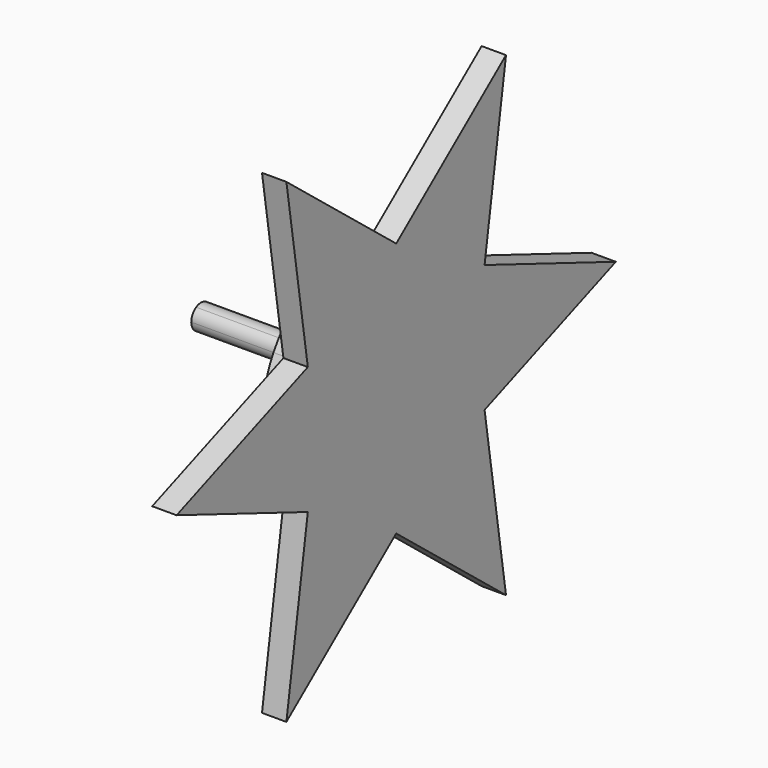
from build123d import *

# Parameters (mm, degrees)
F1_DEPTH = 40.64
F2_DEPTH = 10.16
F3_DEPTH = 5.08


with BuildPart() as f1:
    # F0 (on Right) → F1 (new body)
    with BuildSketch(Plane.YZ):
        with BuildLine():
            Line((-1.27, -2.1997045256), (0, 0))
            Line((0, 0), (-2.54, 0))
            ThreePointArc((-2.54, 0), (-2.1997045256, -1.27), (-1.27, -2.1997045256))
        make_face()
        with BuildLine():
            Line((1.27, -2.1997045256), (0, 0))
            Line((0, 0), (-1.27, -2.1997045256))
            ThreePointArc((-1.27, -2.1997045256), (0, -2.54), (1.27, -2.1997045256))
        make_face()
        with BuildLine():
            ThreePointArc((1.27, -2.1997045256), (2.1997045256, -1.27), (2.54, 0))
            Line((2.54, 0), (0, 0))
            Line((0, 0), (1.27, -2.1997045256))
        make_face()
        with BuildLine():
            Line((0, 0), (2.54, 0))
            ThreePointArc((2.54, 0), (2.1997045256, 1.27), (1.27, 2.1997045256))
            Line((1.27, 2.1997045256), (0, 0))
        make_face()
        with BuildLine():
            Line((-1.27, 2.1997045256), (0, 0))
            Line((0, 0), (1.27, 2.1997045256))
            ThreePointArc((1.27, 2.1997045256), (0, 2.54), (-1.27, 2.1997045256))
        make_face()
        with BuildLine():
            Line((-2.54, 0), (0, 0))
            Line((0, 0), (-1.27, 2.1997045256))
            ThreePointArc((-1.27, 2.1997045256), (-2.1997045256, 1.27), (-2.54, 0))
        make_face()
    extrude(amount=-F1_DEPTH)

    # F0 (on Right) → F2 (join)
    with BuildSketch(Plane.YZ):
        with BuildLine():
            ThreePointArc((21.6980938733, -4.8107532948), (22.0928807689, -2.419761214), (22.225, 0))
            Line((22.225, 0), (20.9576915714, 0))
            Line((20.9576915714, 0), (21.6980938733, -4.8107532948))
        make_face()
        with BuildLine():
            Line((20.9576915714, 0), (22.225, 0))
            ThreePointArc((22.225, 0), (22.0928807689, 2.4197612139), (21.6980938733, 4.8107532948))
            Line((21.6980938733, 4.8107532948), (20.9576915714, 0))
        make_face()
        with BuildLine():
            Line((19.2474145991, -11.1125), (20.9576915714, 0))
            Line((20.9576915714, 0), (2.54, 0))
            ThreePointArc((2.54, 0), (2.1997045256, -1.27), (1.27, -2.1997045256))
            Line((1.27, -2.1997045256), (10.4788457857, -18.1498933056))
            Line((10.4788457857, -18.1498933056), (19.2474145991, -11.1125))
        make_face()
        with BuildLine():
            Line((2.54, 0), (20.9576915714, 0))
            Line((20.9576915714, 0), (19.2474145991, 11.1125))
            Line((19.2474145991, 11.1125), (10.4788457857, 18.1498933056))
            Line((10.4788457857, 18.1498933056), (1.27, 2.1997045256))
            ThreePointArc((1.27, 2.1997045256), (2.1997045256, 1.27), (2.54, 0))
        make_face()
        with BuildLine():
            Line((19.2474145991, 11.1125), (20.9576915714, 0))
            Line((20.9576915714, 0), (21.6980938733, 4.8107532948))
            ThreePointArc((21.6980938733, 4.8107532948), (20.713803825, 8.0553681542), (19.2474145991, 11.1125))
        make_face()
        with BuildLine():
            Line((21.6980938733, -4.8107532948), (20.9576915714, 0))
            Line((20.9576915714, 0), (19.2474145991, -11.1125))
            ThreePointArc((19.2474145991, -11.1125), (20.713803825, -8.0553681542), (21.6980938733, -4.8107532948))
        make_face()
        with BuildLine():
            Line((10.4788457857, 18.1498933056), (11.1125, 19.2474145991))
            ThreePointArc((11.1125, 19.2474145991), (8.9508657021, 20.3428765956), (6.682812372, 21.1964771554))
            Line((6.682812372, 21.1964771554), (10.4788457857, 18.1498933056))
        make_face()
        with BuildLine():
            ThreePointArc((15.0152815013, 16.3857238606), (13.1420150668, 17.9231153816), (11.1125, 19.2474145991))
            Line((11.1125, 19.2474145991), (10.4788457857, 18.1498933056))
            Line((10.4788457857, 18.1498933056), (15.0152815013, 16.3857238606))
        make_face()
        with BuildLine():
            Line((10.4788457857, -18.1498933056), (11.1125, -19.2474145991))
            ThreePointArc((11.1125, -19.2474145991), (13.1420150668, -17.9231153816), (15.0152815013, -16.3857238606))
            Line((15.0152815013, -16.3857238606), (10.4788457857, -18.1498933056))
        make_face()
        with BuildLine():
            ThreePointArc((6.682812372, -21.1964771554), (8.9508657021, -20.3428765956), (11.1125, -19.2474145991))
            Line((11.1125, -19.2474145991), (10.4788457857, -18.1498933056))
            Line((10.4788457857, -18.1498933056), (6.682812372, -21.1964771554))
        make_face()
        with BuildLine():
            ThreePointArc((19.2474145991, 11.1125), (17.3330553708, 13.9109962444), (15.0152815013, 16.3857238606))
            Line((15.0152815013, 16.3857238606), (10.4788457857, 18.1498933056))
            Line((10.4788457857, 18.1498933056), (19.2474145991, 11.1125))
        make_face()
        with BuildLine():
            Line((10.4788457857, -18.1498933056), (15.0152815013, -16.3857238606))
            ThreePointArc((15.0152815013, -16.3857238606), (17.3330553708, -13.9109962444), (19.2474145991, -11.1125))
            Line((19.2474145991, -11.1125), (10.4788457857, -18.1498933056))
        make_face()
        with BuildLine():
            Line((-10.4788457857, 18.1498933056), (-11.1125, 19.2474145991))
            ThreePointArc((-11.1125, 19.2474145991), (-13.1420150668, 17.9231153816), (-15.0152815013, 16.3857238606))
            Line((-15.0152815013, 16.3857238606), (-10.4788457857, 18.1498933056))
        make_face()
        with BuildLine():
            ThreePointArc((-6.682812372, 21.1964771554), (-8.9508657021, 20.3428765956), (-11.1125, 19.2474145991))
            Line((-11.1125, 19.2474145991), (-10.4788457857, 18.1498933056))
            Line((-10.4788457857, 18.1498933056), (-6.682812372, 21.1964771554))
        make_face()
        with BuildLine():
            Line((10.4788457857, 18.1498933056), (6.682812372, 21.1964771554))
            ThreePointArc((6.682812372, 21.1964771554), (3.3807484542, 21.9663643985), (0, 22.225))
            Line((0, 22.225), (10.4788457857, 18.1498933056))
        make_face()
        with BuildLine():
            ThreePointArc((0, 22.225), (-3.3807484542, 21.9663643985), (-6.682812372, 21.1964771554))
            Line((-6.682812372, 21.1964771554), (-10.4788457857, 18.1498933056))
            Line((-10.4788457857, 18.1498933056), (0, 22.225))
        make_face()
        with BuildLine():
            Line((1.27, 2.1997045256), (10.4788457857, 18.1498933056))
            Line((10.4788457857, 18.1498933056), (0, 22.225))
            Line((0, 22.225), (-10.4788457857, 18.1498933056))
            Line((-10.4788457857, 18.1498933056), (-1.27, 2.1997045256))
            ThreePointArc((-1.27, 2.1997045256), (0, 2.54), (1.27, 2.1997045256))
        make_face()
        with BuildLine():
            Line((-10.4788457857, -18.1498933056), (-11.1125, -19.2474145991))
            ThreePointArc((-11.1125, -19.2474145991), (-8.9508657021, -20.3428765956), (-6.682812372, -21.1964771554))
            Line((-6.682812372, -21.1964771554), (-10.4788457857, -18.1498933056))
        make_face()
        with BuildLine():
            ThreePointArc((-15.0152815013, -16.3857238606), (-13.1420150668, -17.9231153816), (-11.1125, -19.2474145991))
            Line((-11.1125, -19.2474145991), (-10.4788457857, -18.1498933056))
            Line((-10.4788457857, -18.1498933056), (-15.0152815013, -16.3857238606))
        make_face()
        with BuildLine():
            Line((-10.4788457857, -18.1498933056), (-6.682812372, -21.1964771554))
            ThreePointArc((-6.682812372, -21.1964771554), (-3.3807484542, -21.9663643985), (0, -22.225))
            Line((0, -22.225), (-10.4788457857, -18.1498933056))
        make_face()
        with BuildLine():
            ThreePointArc((0, -22.225), (3.3807484542, -21.9663643985), (6.682812372, -21.1964771554))
            Line((6.682812372, -21.1964771554), (10.4788457857, -18.1498933056))
            Line((10.4788457857, -18.1498933056), (0, -22.225))
        make_face()
        with BuildLine():
            Line((0, -22.225), (10.4788457857, -18.1498933056))
            Line((10.4788457857, -18.1498933056), (1.27, -2.1997045256))
            ThreePointArc((1.27, -2.1997045256), (0, -2.54), (-1.27, -2.1997045256))
            Line((-1.27, -2.1997045256), (-10.4788457857, -18.1498933056))
            Line((-10.4788457857, -18.1498933056), (0, -22.225))
        make_face()
        with BuildLine():
            ThreePointArc((-21.6980938733, 4.8107532948), (-22.0928807689, 2.419761214), (-22.225, 0))
            Line((-22.225, 0), (-20.9576915714, 0))
            Line((-20.9576915714, 0), (-21.6980938733, 4.8107532948))
        make_face()
        with BuildLine():
            Line((-20.9576915714, 0), (-22.225, 0))
            ThreePointArc((-22.225, 0), (-22.0928807689, -2.419761214), (-21.6980938733, -4.8107532948))
            Line((-21.6980938733, -4.8107532948), (-20.9576915714, 0))
        make_face()
        with BuildLine():
            Line((-10.4788457857, 18.1498933056), (-15.0152815013, 16.3857238606))
            ThreePointArc((-15.0152815013, 16.3857238606), (-17.3330553708, 13.9109962444), (-19.2474145991, 11.1125))
            Line((-19.2474145991, 11.1125), (-10.4788457857, 18.1498933056))
        make_face()
        with BuildLine():
            ThreePointArc((-19.2474145991, 11.1125), (-20.713803825, 8.0553681542), (-21.6980938733, 4.8107532948))
            Line((-21.6980938733, 4.8107532948), (-20.9576915714, 0))
            Line((-20.9576915714, 0), (-19.2474145991, 11.1125))
        make_face()
        with BuildLine():
            Line((-1.27, 2.1997045256), (-10.4788457857, 18.1498933056))
            Line((-10.4788457857, 18.1498933056), (-19.2474145991, 11.1125))
            Line((-19.2474145991, 11.1125), (-20.9576915714, 0))
            Line((-20.9576915714, 0), (-2.54, 0))
            ThreePointArc((-2.54, 0), (-2.1997045256, 1.27), (-1.27, 2.1997045256))
        make_face()
        with BuildLine():
            ThreePointArc((-19.2474145991, -11.1125), (-17.3330553708, -13.9109962444), (-15.0152815013, -16.3857238606))
            Line((-15.0152815013, -16.3857238606), (-10.4788457857, -18.1498933056))
            Line((-10.4788457857, -18.1498933056), (-19.2474145991, -11.1125))
        make_face()
        with BuildLine():
            Line((-20.9576915714, 0), (-21.6980938733, -4.8107532948))
            ThreePointArc((-21.6980938733, -4.8107532948), (-20.713803825, -8.0553681542), (-19.2474145991, -11.1125))
            Line((-19.2474145991, -11.1125), (-20.9576915714, 0))
        make_face()
        with BuildLine():
            Line((-19.2474145991, -11.1125), (-10.4788457857, -18.1498933056))
            Line((-10.4788457857, -18.1498933056), (-1.27, -2.1997045256))
            ThreePointArc((-1.27, -2.1997045256), (-2.1997045256, -1.27), (-2.54, 0))
            Line((-2.54, 0), (-20.9576915714, 0))
            Line((-20.9576915714, 0), (-19.2474145991, -11.1125))
        make_face()
    extrude(amount=-F2_DEPTH)

    # F0 (on Right) → F3 (join)
    with BuildSketch(Plane.YZ):
        with BuildLine():
            Line((23.0015517527, -13.2799520962), (57.15, 0))
            Line((57.15, 0), (22.225, 0))
            ThreePointArc((22.225, 0), (22.0928807689, -2.419761214), (21.6980938733, -4.8107532948))
            Line((21.6980938733, -4.8107532948), (23.0015517527, -13.2799520962))
        make_face()
        with BuildLine():
            Line((22.225, 0), (57.15, 0))
            Line((57.15, 0), (23.0015517527, 13.2799520962))
            Line((23.0015517527, 13.2799520962), (21.6980938733, 4.8107532948))
            ThreePointArc((21.6980938733, 4.8107532948), (22.0928807689, 2.4197612139), (22.225, 0))
        make_face()
        with BuildLine():
            Line((11.1125, 19.2474145991), (28.575, 49.4933518263))
            Line((28.575, 49.4933518263), (0, 26.5599041924))
            Line((0, 26.5599041924), (6.682812372, 21.1964771554))
            ThreePointArc((6.682812372, 21.1964771554), (8.9508657021, 20.3428765956), (11.1125, 19.2474145991))
        make_face()
        with BuildLine():
            Line((23.0015517527, 13.2799520962), (28.575, 49.4933518263))
            Line((28.575, 49.4933518263), (11.1125, 19.2474145991))
            ThreePointArc((11.1125, 19.2474145991), (13.1420150668, 17.9231153816), (15.0152815013, 16.3857238606))
            Line((15.0152815013, 16.3857238606), (23.0015517527, 13.2799520962))
        make_face()
        with BuildLine():
            Line((11.1125, -19.2474145991), (28.575, -49.4933518263))
            Line((28.575, -49.4933518263), (23.0015517527, -13.2799520962))
            Line((23.0015517527, -13.2799520962), (15.0152815013, -16.3857238606))
            ThreePointArc((15.0152815013, -16.3857238606), (13.1420150668, -17.9231153816), (11.1125, -19.2474145991))
        make_face()
        with BuildLine():
            Line((0, -26.5599041924), (28.575, -49.4933518263))
            Line((28.575, -49.4933518263), (11.1125, -19.2474145991))
            ThreePointArc((11.1125, -19.2474145991), (8.9508657021, -20.3428765956), (6.682812372, -21.1964771554))
            Line((6.682812372, -21.1964771554), (0, -26.5599041924))
        make_face()
        with BuildLine():
            Line((21.6980938733, 4.8107532948), (23.0015517527, 13.2799520962))
            Line((23.0015517527, 13.2799520962), (15.0152815013, 16.3857238606))
            ThreePointArc((15.0152815013, 16.3857238606), (17.3330553708, 13.9109962444), (19.2474145991, 11.1125))
            ThreePointArc((19.2474145991, 11.1125), (20.713803825, 8.0553681542), (21.6980938733, 4.8107532948))
        make_face()
        with BuildLine():
            Line((15.0152815013, -16.3857238606), (23.0015517527, -13.2799520962))
            Line((23.0015517527, -13.2799520962), (21.6980938733, -4.8107532948))
            ThreePointArc((21.6980938733, -4.8107532948), (20.713803825, -8.0553681542), (19.2474145991, -11.1125))
            ThreePointArc((19.2474145991, -11.1125), (17.3330553708, -13.9109962444), (15.0152815013, -16.3857238606))
        make_face()
        with BuildLine():
            Line((-11.1125, 19.2474145991), (-28.575, 49.4933518263))
            Line((-28.575, 49.4933518263), (-23.0015517527, 13.2799520962))
            Line((-23.0015517527, 13.2799520962), (-15.0152815013, 16.3857238606))
            ThreePointArc((-15.0152815013, 16.3857238606), (-13.1420150668, 17.9231153816), (-11.1125, 19.2474145991))
        make_face()
        with BuildLine():
            Line((0, 26.5599041924), (-28.575, 49.4933518263))
            Line((-28.575, 49.4933518263), (-11.1125, 19.2474145991))
            ThreePointArc((-11.1125, 19.2474145991), (-8.9508657021, 20.3428765956), (-6.682812372, 21.1964771554))
            Line((-6.682812372, 21.1964771554), (0, 26.5599041924))
        make_face()
        with BuildLine():
            Line((6.682812372, 21.1964771554), (0, 26.5599041924))
            Line((0, 26.5599041924), (-6.682812372, 21.1964771554))
            ThreePointArc((-6.682812372, 21.1964771554), (-3.3807484542, 21.9663643985), (0, 22.225))
            ThreePointArc((0, 22.225), (3.3807484542, 21.9663643985), (6.682812372, 21.1964771554))
        make_face()
        with BuildLine():
            Line((-11.1125, -19.2474145991), (-28.575, -49.4933518263))
            Line((-28.575, -49.4933518263), (0, -26.5599041924))
            Line((0, -26.5599041924), (-6.682812372, -21.1964771554))
            ThreePointArc((-6.682812372, -21.1964771554), (-8.9508657021, -20.3428765956), (-11.1125, -19.2474145991))
        make_face()
        with BuildLine():
            Line((-23.0015517527, -13.2799520962), (-28.575, -49.4933518263))
            Line((-28.575, -49.4933518263), (-11.1125, -19.2474145991))
            ThreePointArc((-11.1125, -19.2474145991), (-13.1420150668, -17.9231153816), (-15.0152815013, -16.3857238606))
            Line((-15.0152815013, -16.3857238606), (-23.0015517527, -13.2799520962))
        make_face()
        with BuildLine():
            Line((-6.682812372, -21.1964771554), (0, -26.5599041924))
            Line((0, -26.5599041924), (6.682812372, -21.1964771554))
            ThreePointArc((6.682812372, -21.1964771554), (3.3807484542, -21.9663643985), (0, -22.225))
            ThreePointArc((0, -22.225), (-3.3807484542, -21.9663643985), (-6.682812372, -21.1964771554))
        make_face()
        with BuildLine():
            Line((10.4788457857, -18.1498933056), (15.0152815013, -16.3857238606))
            ThreePointArc((15.0152815013, -16.3857238606), (17.3330553708, -13.9109962444), (19.2474145991, -11.1125))
            Line((19.2474145991, -11.1125), (10.4788457857, -18.1498933056))
        make_face()
        with BuildLine():
            Line((-23.0015517527, 13.2799520962), (-57.15, 0))
            Line((-57.15, 0), (-22.225, 0))
            ThreePointArc((-22.225, 0), (-22.0928807689, 2.419761214), (-21.6980938733, 4.8107532948))
            Line((-21.6980938733, 4.8107532948), (-23.0015517527, 13.2799520962))
        make_face()
        with BuildLine():
            Line((-22.225, 0), (-57.15, 0))
            Line((-57.15, 0), (-23.0015517527, -13.2799520962))
            Line((-23.0015517527, -13.2799520962), (-21.6980938733, -4.8107532948))
            ThreePointArc((-21.6980938733, -4.8107532948), (-22.0928807689, -2.419761214), (-22.225, 0))
        make_face()
        with BuildLine():
            Line((-15.0152815013, 16.3857238606), (-23.0015517527, 13.2799520962))
            Line((-23.0015517527, 13.2799520962), (-21.6980938733, 4.8107532948))
            ThreePointArc((-21.6980938733, 4.8107532948), (-20.713803825, 8.0553681542), (-19.2474145991, 11.1125))
            ThreePointArc((-19.2474145991, 11.1125), (-17.3330553708, 13.9109962444), (-15.0152815013, 16.3857238606))
        make_face()
        with BuildLine():
            Line((1.27, 2.1997045256), (10.4788457857, 18.1498933056))
            Line((10.4788457857, 18.1498933056), (0, 22.225))
            Line((0, 22.225), (-10.4788457857, 18.1498933056))
            Line((-10.4788457857, 18.1498933056), (-1.27, 2.1997045256))
            ThreePointArc((-1.27, 2.1997045256), (0, 2.54), (1.27, 2.1997045256))
        make_face()
        with BuildLine():
            Line((-21.6980938733, -4.8107532948), (-23.0015517527, -13.2799520962))
            Line((-23.0015517527, -13.2799520962), (-15.0152815013, -16.3857238606))
            ThreePointArc((-15.0152815013, -16.3857238606), (-17.3330553708, -13.9109962444), (-19.2474145991, -11.1125))
            ThreePointArc((-19.2474145991, -11.1125), (-20.713803825, -8.0553681542), (-21.6980938733, -4.8107532948))
        make_face()
        with BuildLine():
            Line((-10.4788457857, -18.1498933056), (-6.682812372, -21.1964771554))
            ThreePointArc((-6.682812372, -21.1964771554), (-3.3807484542, -21.9663643985), (0, -22.225))
            Line((0, -22.225), (-10.4788457857, -18.1498933056))
        make_face()
        with BuildLine():
            Line((0, -22.225), (10.4788457857, -18.1498933056))
            Line((10.4788457857, -18.1498933056), (1.27, -2.1997045256))
            ThreePointArc((1.27, -2.1997045256), (0, -2.54), (-1.27, -2.1997045256))
            Line((-1.27, -2.1997045256), (-10.4788457857, -18.1498933056))
            Line((-10.4788457857, -18.1498933056), (0, -22.225))
        make_face()
        with BuildLine():
            Line((-10.4788457857, 18.1498933056), (-15.0152815013, 16.3857238606))
            ThreePointArc((-15.0152815013, 16.3857238606), (-17.3330553708, 13.9109962444), (-19.2474145991, 11.1125))
            Line((-19.2474145991, 11.1125), (-10.4788457857, 18.1498933056))
        make_face()
        with BuildLine():
            Line((-20.9576915714, 0), (-21.6980938733, -4.8107532948))
            ThreePointArc((-21.6980938733, -4.8107532948), (-20.713803825, -8.0553681542), (-19.2474145991, -11.1125))
            Line((-19.2474145991, -11.1125), (-20.9576915714, 0))
        make_face()
        with BuildLine():
            Line((-19.2474145991, -11.1125), (-10.4788457857, -18.1498933056))
            Line((-10.4788457857, -18.1498933056), (-1.27, -2.1997045256))
            ThreePointArc((-1.27, -2.1997045256), (-2.1997045256, -1.27), (-2.54, 0))
            Line((-2.54, 0), (-20.9576915714, 0))
            Line((-20.9576915714, 0), (-19.2474145991, -11.1125))
        make_face()
    extrude(amount=-F3_DEPTH)


solid = f1.part
